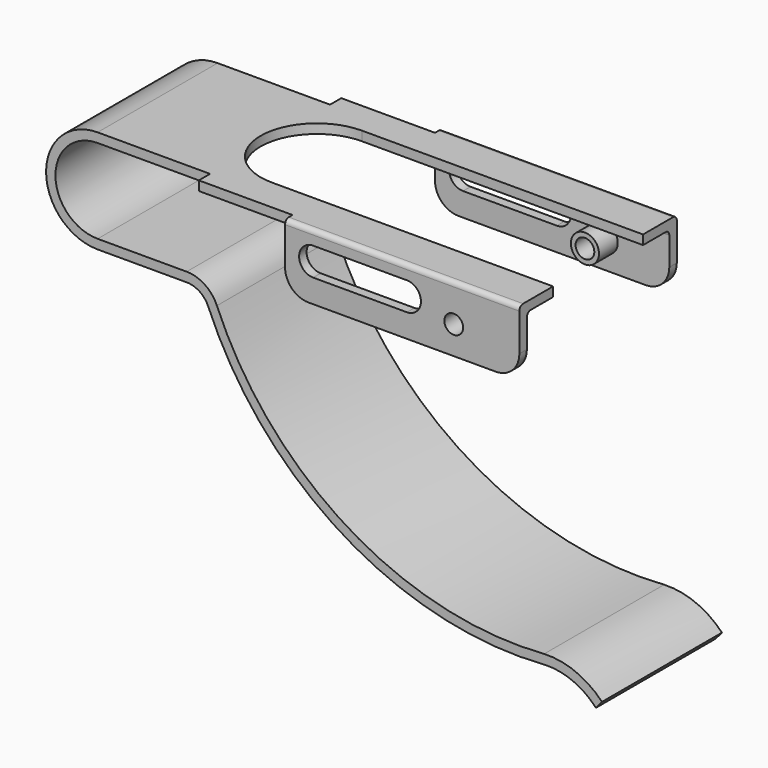
from build123d import *

# Parameters (mm, degrees)
F1_DEPTH  = 16
F2_W      = 70
F2_H      = 3
F3_DEPTH  = 2
F4_W      = 50
F4_H      = 14
F5_DEPTH  = 2
F6_R      = 1
F9_DEPTH  = 2
F11_DEPTH = 42.001
F13_D     = 4
F14_R     = 3
F14_R_2   = 2
F15_DEPTH = 5
F17_R     = 5


with BuildPart() as f1:
    # F0 (on Front) → F1 (new body)
    with BuildSketch(Plane.XZ):
        with BuildLine():
            Line((94, 11), (0, 11))
            ThreePointArc((0, 11), (-11, 0), (0, -11))
            Line((0, -11), (19, -11))
            ThreePointArc((19, -11), (21.7681124643, -11.8361612201), (23.6103896104, -14.064978646))
            ThreePointArc((23.6103896104, -14.064978646), (52.4237101957, -47.6174640031), (95.4149528414, -57.9967593826))
            ThreePointArc((95.4149528414, -57.9967593826), (101.3804745105, -59.0597282402), (106.3380534538, -62.5439444501))
            Line((106.3380534538, -62.5439444501), (107.6335766724, -61))
            ThreePointArc((107.6335766724, -61), (102.0097459375, -57.1560789275), (95.2965735981, -56))
            ThreePointArc((95.2965735981, -56), (53.4811996085, -45.9198240056), (25.4545454545, -13.2909701044))
            ThreePointArc((25.4545454545, -13.2909701044), (22.87535745, -10.1706257081), (19, -9))
            Line((19, -9), (0, -9))
            ThreePointArc((0, -9), (-9, 0), (0, 9))
            Line((0, 9), (94, 9))
            Line((94, 9), (94, 11))
        make_face()
    extrude(amount=F1_DEPTH)

    # F2 (on face) → F3 (join)
    with BuildSketch(Plane.XY.offset(11)):
        with Locations((59, -17.5)):
            Rectangle(F2_W, F2_H)
    extrude(amount=-F3_DEPTH)

    # F4 (on face) → F5 (join)
    with BuildSketch(Plane.XZ.offset(19)):
        with Locations((69, 4)):
            Rectangle(F4_W, F4_H)
    extrude(amount=F5_DEPTH)

    # F6
    f6_edges = [f1.edges().sort_by_distance(p)[0] for p in [
        (69, -21, 11),
        (69, -19, 9),
    ]]
    fillet(f6_edges, radius=F6_R)

    # F7: F1 across plane


with BuildPart() as f1_1:
    add(f1.part)
    add(f1.part.mirror(Plane.XZ))

    # F8 (on face) → F9 (cut)
    with BuildSketch(Plane.XY.offset(11)):
        with BuildLine():
            Line((94, 12), (34, 12))
            ThreePointArc((34, 12), (22, 0), (34, -12))
            Line((34, -12), (94, -12))
            Line((94, -12), (94, 12))
        make_face()
    extrude(amount=-F9_DEPTH, mode=Mode.SUBTRACT)

    # F10 (on face) → F11 (cut, through all)
    with BuildSketch(Plane(origin=(0, 21, 0), x_dir=(-1, 0, 0), z_dir=(0, 1, 0))):
        with BuildLine():
            ThreePointArc((-70, 8), (-73, 5), (-70, 2))
            Line((-70, 2), (-50, 2))
            ThreePointArc((-50, 2), (-47, 5), (-50, 8))
            Line((-50, 8), (-70, 8))
        make_face()
    extrude(amount=-F11_DEPTH, mode=Mode.SUBTRACT)

    # F13 (through all)
    with Locations(Plane(origin=(0, 21, 0), x_dir=(-1, 0, 0), z_dir=(0, 1, 0))):
        with Locations((-80, 3)):
            Hole(F13_D / 2)

    # F14 (on face) → F15 (join)
    with BuildSketch(Plane.XZ.offset(-19)):
        with Locations((80, 3)):
            Circle(F14_R)
        with Locations((80, 3)):
            Circle(F14_R_2, mode=Mode.SUBTRACT)
    extrude(amount=F15_DEPTH)

    # F16: F1 across plane


with BuildPart() as f1_2:
    add(f1_1.part)
    add(f1_1.part.mirror(Plane.XZ))

    # F17
    f17_edges = [f1_2.edges().sort_by_distance(p)[0] for p in [
        (94, 20, -3),
        (44, 20, -3),
        (94, -20, -3),
        (44, -20, -3),
    ]]
    fillet(f17_edges, radius=F17_R)


solid = f1_2.part
